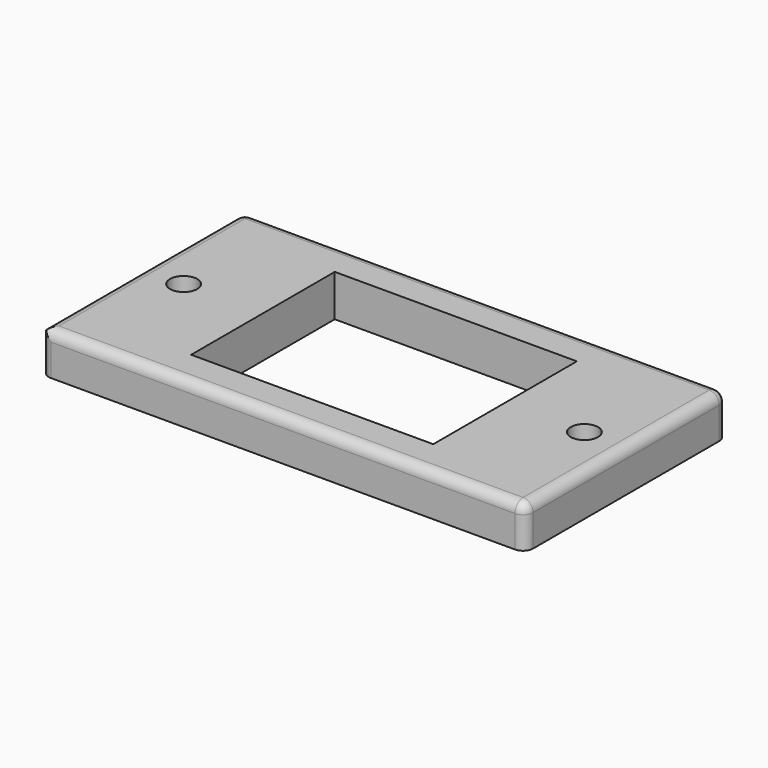
from build123d import *

# Parameters (mm, degrees)
F0_W         = 57.9988658428
F0_H         = 30.2602835
F1_DEPTH     = 5
F3_D         = 3.2639
F4_W         = 29
F4_H         = 21.5
F5_DEPTH     = 25
F7_R         = 1.207
F8_R         = 1.207
F9_T1_DEPTH  = 6.8105
F9_T3_DEPTH  = 32.0707835
F9_T6_ANGLE  = 90
F9_T7_DEPTH  = 9.828
F9_T9_DEPTH  = 58.6023658428
F9_T11_DEPTH = 6.8105
F9_T14_ANGLE = 90


# Not quite as in the source:
# - a fillet or chamfer that OpenCascade refuses, or shapes differently, is made with other operations: its cross-section is extruded or revolved along the edge and cut away or added
# - a feature of the source that left no trace in its solid (it failed there, or was rolled back) is left out


with BuildPart() as f1:
    # F0 (on Top) → F1 (new body)
    with BuildSketch(Plane.XY):
        Rectangle(F0_W, F0_H)
    extrude(amount=-F1_DEPTH)

    # F3 (through all)
    with Locations(Plane.XY):
        with Locations((-23.9994329214, 0), (23.9994329214, 0)):
            Hole(F3_D / 2)

    # F4 (on Top) → F5 (cut)
    with BuildSketch(Plane.XY):
        Rectangle(F4_W, F4_H)
    extrude(amount=-F5_DEPTH, mode=Mode.SUBTRACT)

    # F7
    f7_edges = [f1.edges().sort_by_distance(p)[0] for p in [
        (0, 15.130142, 0),
    ]]
    fillet(f7_edges, radius=F7_R)

    # F8
    f8_edges = [f1.edges().sort_by_distance(p)[0] for p in [
        (28.999433, -0.6035, 0),
    ]]
    fillet(f8_edges, radius=F8_R)

    # F9: fillet of radius 1.207 on 7 edges, made by hand

    # F9_s2 → F9_t1 (cut)
    with BuildSketch(Plane.XY.offset(-8.0175)):
        with BuildLine():
            ThreePointArc((-27.7924329214, 15.13014175), (-28.6459108063, 14.7766196349), (-28.9994329214, 13.92314175))
            Line((-28.9994329214, 13.92314175), (-28.9994329214, 15.13014175))
            Line((-28.9994329214, 15.13014175), (-27.7924329214, 15.13014175))
        make_face()
    extrude(amount=F9_T1_DEPTH, mode=Mode.SUBTRACT)

    # F9_s4 → F9_t3 (cut)
    with BuildSketch(Plane.XZ.offset(-13.92314175)):
        with BuildLine():
            ThreePointArc((-28.9994329214, -1.207), (-28.6459108063, -0.3535221151), (-27.7924329214, 0))
            Line((-27.7924329214, 0), (-28.9994329214, 0))
            Line((-28.9994329214, 0), (-28.9994329214, -1.207))
        make_face()
    extrude(amount=F9_T3_DEPTH, mode=Mode.SUBTRACT)

    # F9_s5 → F9_t6 (revolve, cut)
    with BuildSketch(Plane.XY.offset(-1.207)):
        with BuildLine():
            ThreePointArc((-27.7924329214, 15.13014175), (-28.6459108063, 14.7766196349), (-28.9994329214, 13.92314175))
            Line((-28.9994329214, 13.92314175), (-28.9994329214, 15.13014175))
            Line((-28.9994329214, 15.13014175), (-27.7924329214, 15.13014175))
        make_face()
    revolve(axis=Axis((-28.9994329214, 13.92314175, -1.207), (1, 0, 0)), revolution_arc=F9_T6_ANGLE, mode=Mode.SUBTRACT)

    # F9_s8 → F9_t7 (cut)
    with BuildSketch(Plane.XY.offset(-8.0175)):
        with BuildLine():
            ThreePointArc((-28.9994329214, -13.92314175), (-28.6459108063, -14.7766196349), (-27.7924329214, -15.13014175))
            Line((-27.7924329214, -15.13014175), (-28.9994329214, -15.13014175))
            Line((-28.9994329214, -15.13014175), (-28.9994329214, -13.92314175))
        make_face()
    extrude(amount=F9_T7_DEPTH, mode=Mode.SUBTRACT)

    # F9_s10 → F9_t9 (cut)
    with BuildSketch(Plane.YZ.offset(-30.8099329214)):
        with BuildLine():
            ThreePointArc((-13.92314175, 0), (-14.7766196349, -0.3535221151), (-15.13014175, -1.207))
            Line((-15.13014175, -1.207), (-15.13014175, 0))
            Line((-15.13014175, 0), (-13.92314175, 0))
        make_face()
    extrude(amount=F9_T9_DEPTH, mode=Mode.SUBTRACT)

    # F9_s12 → F9_t11 (cut)
    with BuildSketch(Plane.XY.offset(-8.0175)):
        with BuildLine():
            ThreePointArc((28.9994329214, -13.92314175), (28.6459108063, -14.7766196349), (27.7924329214, -15.13014175))
            Line((27.7924329214, -15.13014175), (28.9994329214, -15.13014175))
            Line((28.9994329214, -15.13014175), (28.9994329214, -13.92314175))
        make_face()
    extrude(amount=F9_T11_DEPTH, mode=Mode.SUBTRACT)

    # F9_s13 → F9_t14 (revolve, cut)
    with BuildSketch(Plane.XY.offset(-1.207)):
        with BuildLine():
            ThreePointArc((27.7924329214, -15.13014175), (28.6459108063, -14.7766196349), (28.9994329214, -13.92314175))
            Line((28.9994329214, -13.92314175), (28.9994329214, -15.13014175))
            Line((28.9994329214, -15.13014175), (27.7924329214, -15.13014175))
        make_face()
    revolve(axis=Axis((27.7924329214, -15.13014175, -1.207), (0, -1, 0)), revolution_arc=F9_T14_ANGLE, mode=Mode.SUBTRACT)


solid = f1.part
